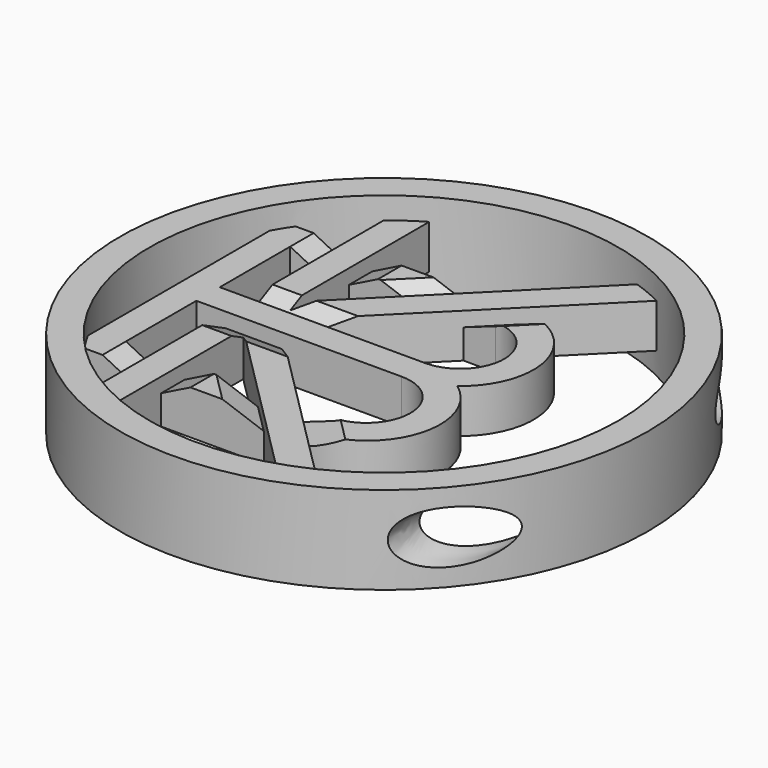
from build123d import *
from build123d import SkipClean  # not in build123d's __all__

# Parameters (mm, degrees)
F1_R          = 9
F1_R_2        = 8
F2_DEPTH      = 2.25
F2_DEPTH_BACK = 0.75
F0_W          = 1
F0_H          = 3
F3_DEPTH      = 1.5
F7_DEPTH      = 25
F7_DEPTH_BACK = 25
F9_DEPTH      = 1
F11_DEPTH     = 1
F13_DEPTH     = 1
F15_DEPTH     = 1
F17_DEPTH     = 3
F19_DEPTH     = 3
F21_DEPTH     = 5
F23_DEPTH     = 5


with BuildPart() as f2:
    # F1 (on Top) → F2 (new body, two sides)
    with BuildSketch(Plane.XY) as f2_sk:
        Circle(F1_R)
        Circle(F1_R_2, mode=Mode.SUBTRACT)
    extrude(amount=F2_DEPTH)
    extrude(f2_sk.sketch, amount=-F2_DEPTH_BACK)

    # F0 (on Top) → F3 (join)
    with BuildSketch(Plane.XY):
        with BuildLine():
            Line((0.9142135624, 4.5), (3.5723219592, 7.1581083968))
            ThreePointArc((3.5723219592, 7.1581083968), (3.080425721, 7.3831549745), (2.5744457825, 7.5744457825))
            Line((2.5744457825, 7.5744457825), (-0.5, 4.5))
            Line((-0.5, 4.5), (0.9142135624, 4.5))
        make_face()
        with BuildLine():
            ThreePointArc((2.5744457825, -7.5744457825), (3.080425721, -7.3831549745), (3.5723219592, -7.1581083968))
            Line((3.5723219592, -7.1581083968), (0.9126884353, -4.4984748729))
            Line((0.9126884353, -4.4984748729), (1, -4.5))
            ThreePointArc((1, -4.5), (3.4017548158, -2.8005849386), (2.5, 0))
            ThreePointArc((2.5, 0), (3.3717082451, 2.790569415), (1, 4.5))
            Line((1, 4.5), (0.9142135624, 4.5))
            Line((0.9142135624, 4.5), (-0.5, 4.5))
            Line((-0.5, 4.5), (-4, 4.5))
            Line((-4, 4.5), (-4, 6.9282032303))
            ThreePointArc((-4, 6.9282032303), (-4.5129471908, 6.6055512755), (-5, 6.2449979984))
            Line((-5, 6.2449979984), (-5, 4.5))
            Line((-5, 4.5), (-6.6143782777, 4.5))
            ThreePointArc((-6.6143782777, 4.5), (-6.814404702, 4.190929319), (-7, 3.8729833462))
            Line((-7, 3.8729833462), (-7, -3.8729833462))
            ThreePointArc((-7, -3.8729833462), (-6.814404702, -4.190929319), (-6.6143782777, -4.5))
            Line((-6.6143782777, -4.5), (-5, -4.5))
            Line((-5, -4.5), (-5, -6.2449979984))
            ThreePointArc((-5, -6.2449979984), (-4.5129471908, -6.6055512755), (-4, -6.9282032303))
            Line((-4, -6.9282032303), (-4, -4.5))
            Line((-4, -4.5), (-0.5, -4.5))
            Line((-0.5, -4.5), (2.5744457825, -7.5744457825))
        make_face()
        with Locations((-5.5, -2)):
            Rectangle(F0_W, F0_H, mode=Mode.SUBTRACT)
        Polygon((-4, -3.5), (-4, -1), (-1.5, -3.5), align=None, mode=Mode.SUBTRACT)
        with BuildLine():
            Line((-3.0857864376, -0.5), (1, -0.5))
            ThreePointArc((1, -0.5), (2.5, -2), (1, -3.5))
            Line((1, -3.5), (-0.0857864376, -3.5))
            Line((-0.0857864376, -3.5), (-3.0857864376, -0.5))
        make_face(mode=Mode.SUBTRACT)
        with Locations((-5.5, 2)):
            Rectangle(F0_W, F0_H, mode=Mode.SUBTRACT)
        Polygon((-4, 3.5), (-1.5, 3.5), (-4, 1), align=None, mode=Mode.SUBTRACT)
        with BuildLine():
            Line((-0.0857864376, 3.5), (1, 3.5))
            ThreePointArc((1, 3.5), (2.5, 2), (1, 0.5))
            Line((1, 0.5), (-3.0857864376, 0.5))
            Line((-3.0857864376, 0.5), (-0.0857864376, 3.5))
        make_face(mode=Mode.SUBTRACT)
    extrude(amount=F3_DEPTH)

    # F6 (on Front) → F7 (cut, two sides)
    with BuildSketch(Plane.XZ) as f7_sk:
        with BuildLine():
            add(Edge.make_bspline(
                [(8, 0.75), (8, 2.3088457268), (6.275, 1.5294228634), (4.55, 0.75), (6.275, -0.0294228634), (8, -0.8088457268), (8, 0.75)],
                knots=[0, 0, 0, 2.0943951024, 2.0943951024, 4.1887902048, 4.1887902048, 6.2831853072, 6.2831853072, 6.2831853072], degree=2, weights=[1, 0.5, 1, 0.5, 1, 0.5, 1]))
        make_face()
    with SkipClean():  # cleaning this boolean's faces spoils the solid; the shape is the same uncleaned
        extrude(amount=F7_DEPTH, mode=Mode.SUBTRACT)
        extrude(f7_sk.sketch, amount=-F7_DEPTH_BACK, mode=Mode.SUBTRACT)

    # F8 (on face) → F9 (cut)
    with BuildSketch(Plane.XZ.offset(-3.5)):
        Polygon((-4, 1.5), (-4, 1), (-3, 1.5), align=None)
    extrude(amount=-F9_DEPTH, mode=Mode.SUBTRACT)

    # F10 (on face) → F11 (cut)
    with BuildSketch(Plane.XZ.offset(-3.5)):
        Polygon((-6, 1.5), (-5, 1), (-5, 1.5), align=None)
    extrude(amount=-F11_DEPTH, mode=Mode.SUBTRACT)

    # F12 (on face) → F13 (cut)
    with BuildSketch(Plane(origin=(0, -3.5, 0), x_dir=(-1, 0, 0), z_dir=(0, 1, 0))):
        Polygon((5, 1.5), (5, 1), (6, 1.5), align=None)
    extrude(amount=-F13_DEPTH, mode=Mode.SUBTRACT)

    # F14 (on face) → F15 (cut)
    with BuildSketch(Plane(origin=(0, -3.5, 0), x_dir=(-1, 0, 0), z_dir=(0, 1, 0))):
        Polygon((3, 1.5), (4, 1), (4, 1.5), align=None)
    extrude(amount=-F15_DEPTH, mode=Mode.SUBTRACT)

    # F16 (on face) → F17 (cut)
    with BuildSketch(Plane(origin=(-5, 0, 0), x_dir=(0, -1, 0), z_dir=(-1, 0, 0))):
        Polygon((-0.5, 1.5), (-1.5, 1.5), (-0.5, 1), align=None)
    extrude(amount=-F17_DEPTH, mode=Mode.SUBTRACT)

    # F18 (on face) → F19 (cut)
    with BuildSketch(Plane(origin=(-5, 0, 0), x_dir=(0, -1, 0), z_dir=(-1, 0, 0))):
        Polygon((0.5, 1.5), (0.5, 1), (1.5, 1.5), align=None)
    extrude(amount=-F19_DEPTH, mode=Mode.SUBTRACT)

    # F20 (on face) → F21 (cut)
    with BuildSketch(Plane(origin=(0.2071067812, 0.2071067812, 0), x_dir=(0.7071067812, -0.7071067812, 0), z_dir=(-0.7071067812, -0.7071067812, 0))):
        Polygon((-3.5355339059, 1.5), (-4.5355339059, 1.5), (-3.5355339059, 1), align=None)
        Polygon((-2.5355339059, 1), (-1.5355339059, 1.5), (-2.5355339059, 1.5), align=None)
    extrude(amount=-F21_DEPTH, mode=Mode.SUBTRACT)

    # F22 (on face) → F23 (cut)
    with BuildSketch(Plane(origin=(0.2071067812, -0.2071067812, 0), x_dir=(0.7071067812, 0.7071067812, 0), z_dir=(0.7071067812, -0.7071067812, 0))):
        Polygon((-2.5355339059, 1), (-1.5355339059, 1.5), (-2.5355339059, 1.5), align=None)
        Polygon((-3.5355339059, 1.5), (-4.5355339059, 1.5), (-3.5355339059, 1), align=None)
    extrude(amount=F23_DEPTH, mode=Mode.SUBTRACT)


solid = f2.part
